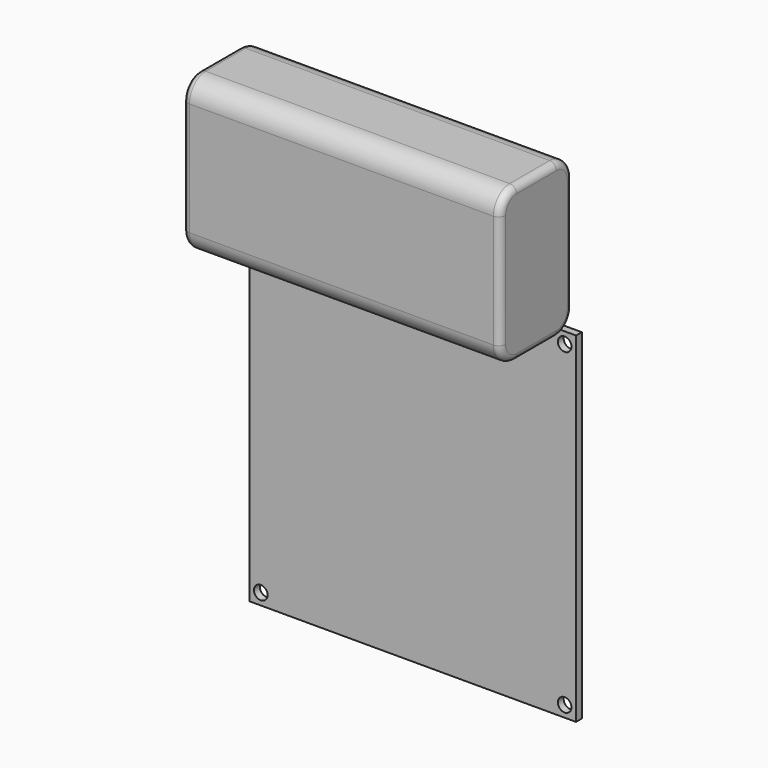
from build123d import *

# Parameters (mm, degrees)
F0_W         = 72
F0_H         = 75
F0_R         = 1.5
F1_DEPTH     = 1.6
F2_W         = 70
F2_H         = 34
F3_DEPTH     = 20
F4_R         = 1.5
F5_T1_DEPTH  = 70
F5_T4_ANGLE  = 90
F5_T6_ANGLE  = 90
F5_T8_ANGLE  = 90
F5_T10_ANGLE = 90
F5_T12_ANGLE = 90
F5_T14_ANGLE = 90
F5_T16_ANGLE = 90
F5_T18_ANGLE = 90


# Not quite as in the source:
# - a fillet or chamfer that OpenCascade refuses, or shapes differently, is made with other operations: its cross-section is extruded or revolved along the edge and cut away or added


with BuildPart() as f1:
    # F0 (on Front) → F1 (new body)
    with BuildSketch(Plane.XZ):
        with Locations((36, -37.5)):
            Rectangle(F0_W, F0_H)
        with Locations((2.5, -72.5)):
            Circle(F0_R, mode=Mode.SUBTRACT)
        with Locations((69.5, -72.5)):
            Circle(F0_R, mode=Mode.SUBTRACT)
        with Locations((2.5, -2.5)):
            Circle(F0_R, mode=Mode.SUBTRACT)
        with Locations((69.5, -2.5)):
            Circle(F0_R, mode=Mode.SUBTRACT)
    extrude(amount=F1_DEPTH)


with BuildPart() as f3:
    # F2 (on Front) → F3 (new body)
    with BuildSketch(Plane.XZ):
        with Locations((35, 17)):
            Rectangle(F2_W, F2_H)
    extrude(amount=F3_DEPTH)

    # F4
    f4_edges = [f3.edges().sort_by_distance(p)[0] for p in [
        (70, -10, 0),
        (70, -10, 34),
        (70, 0, 17),
        (70, -20, 17),
        (0, -10, 34),
        (0, -10, 0),
        (0, 0, 17),
        (0, -20, 17),
    ]]
    fillet(f4_edges, radius=F4_R)

    # F5: fillet of radius 4.5 on 4 edges, made by hand

    # F5_s2 → F5_t1 (cut)
    with BuildSketch(Plane.YZ):
        with BuildLine():
            ThreePointArc((-4.5, 34), (-1.3180194847, 32.6819805153), (0, 29.5))
            Line((0, 29.5), (0, 34))
            Line((0, 34), (-4.5, 34))
        make_face()
        with BuildLine():
            ThreePointArc((0, 4.5), (-1.3180194847, 1.3180194847), (-4.5, 0))
            Line((-4.5, 0), (0, 0))
            Line((0, 0), (0, 4.5))
        make_face()
        with BuildLine():
            ThreePointArc((-15.5, 34), (-18.6819805153, 32.6819805153), (-20, 29.5))
            Line((-20, 29.5), (-20, 34))
            Line((-20, 34), (-15.5, 34))
        make_face()
        with BuildLine():
            ThreePointArc((-20, 4.5), (-18.6819805153, 1.3180194847), (-15.5, 0))
            Line((-15.5, 0), (-20, 0))
            Line((-20, 0), (-20, 4.5))
        make_face()
    extrude(amount=F5_T1_DEPTH, mode=Mode.SUBTRACT)

    # F5_s3 → F5_t4 (revolve, cut)
    with BuildSketch(Plane.XZ.offset(15.5)):
        with BuildLine():
            ThreePointArc((0, 1.5), (0.4393398282, 0.4393398282), (1.5, 0))
            Line((1.5, 0), (0, 0))
            Line((0, 0), (0, 1.5))
        make_face()
    revolve(axis=Axis((0, -15.5, 4.5), (-1, 0, 0)), revolution_arc=F5_T4_ANGLE, mode=Mode.SUBTRACT)

    # F5_s5 → F5_t6 (revolve, cut)
    with BuildSketch(Plane.XY.offset(4.5)):
        with BuildLine():
            ThreePointArc((70, -18.5), (69.5606601718, -19.5606601718), (68.5, -20))
            Line((68.5, -20), (70, -20))
            Line((70, -20), (70, -18.5))
        make_face()
    revolve(axis=Axis((70, -15.5, 4.5), (1, 0, 0)), revolution_arc=F5_T6_ANGLE, mode=Mode.SUBTRACT)

    # F5_s7 → F5_t8 (revolve, cut)
    with BuildSketch(Plane.XZ.offset(15.5)):
        with BuildLine():
            ThreePointArc((70, 32.5), (69.5606601718, 33.5606601718), (68.5, 34))
            Line((68.5, 34), (70, 34))
            Line((70, 34), (70, 32.5))
        make_face()
    revolve(axis=Axis((70, -15.5, 29.5), (1, 0, 0)), revolution_arc=F5_T8_ANGLE, mode=Mode.SUBTRACT)

    # F5_s9 → F5_t10 (revolve, cut)
    with BuildSketch(Plane.XY.offset(29.5)):
        with BuildLine():
            ThreePointArc((0, -18.5), (0.4393398282, -19.5606601718), (1.5, -20))
            Line((1.5, -20), (0, -20))
            Line((0, -20), (0, -18.5))
        make_face()
    revolve(axis=Axis((0, -15.5, 29.5), (-1, 0, 0)), revolution_arc=F5_T10_ANGLE, mode=Mode.SUBTRACT)

    # F5_s11 → F5_t12 (revolve, cut)
    with BuildSketch(Plane.XY.offset(4.5)):
        with BuildLine():
            ThreePointArc((0, -1.5), (0.4393398282, -0.4393398282), (1.5, 0))
            Line((1.5, 0), (0, 0))
            Line((0, 0), (0, -1.5))
        make_face()
    revolve(axis=Axis((0, -4.5, 4.5), (-1, 0, 0)), revolution_arc=F5_T12_ANGLE, mode=Mode.SUBTRACT)

    # F5_s13 → F5_t14 (revolve, cut)
    with BuildSketch(Plane.XZ.offset(4.5)):
        with BuildLine():
            ThreePointArc((70, 1.5), (69.5606601718, 0.4393398282), (68.5, 0))
            Line((68.5, 0), (70, 0))
            Line((70, 0), (70, 1.5))
        make_face()
    revolve(axis=Axis((70, -4.5, 4.5), (1, 0, 0)), revolution_arc=F5_T14_ANGLE, mode=Mode.SUBTRACT)

    # F5_s15 → F5_t16 (revolve, cut)
    with BuildSketch(Plane.XY.offset(29.5)):
        with BuildLine():
            ThreePointArc((70, -1.5), (69.5606601718, -0.4393398282), (68.5, 0))
            Line((68.5, 0), (70, 0))
            Line((70, 0), (70, -1.5))
        make_face()
    revolve(axis=Axis((70, -4.5, 29.5), (1, 0, 0)), revolution_arc=F5_T16_ANGLE, mode=Mode.SUBTRACT)

    # F5_s17 → F5_t18 (revolve, cut)
    with BuildSketch(Plane.XZ.offset(4.5)):
        with BuildLine():
            ThreePointArc((0, 32.5), (0.4393398282, 33.5606601718), (1.5, 34))
            Line((1.5, 34), (0, 34))
            Line((0, 34), (0, 32.5))
        make_face()
    revolve(axis=Axis((0, -4.5, 29.5), (-1, 0, 0)), revolution_arc=F5_T18_ANGLE, mode=Mode.SUBTRACT)


solid = Compound([f1.part, f3.part])
